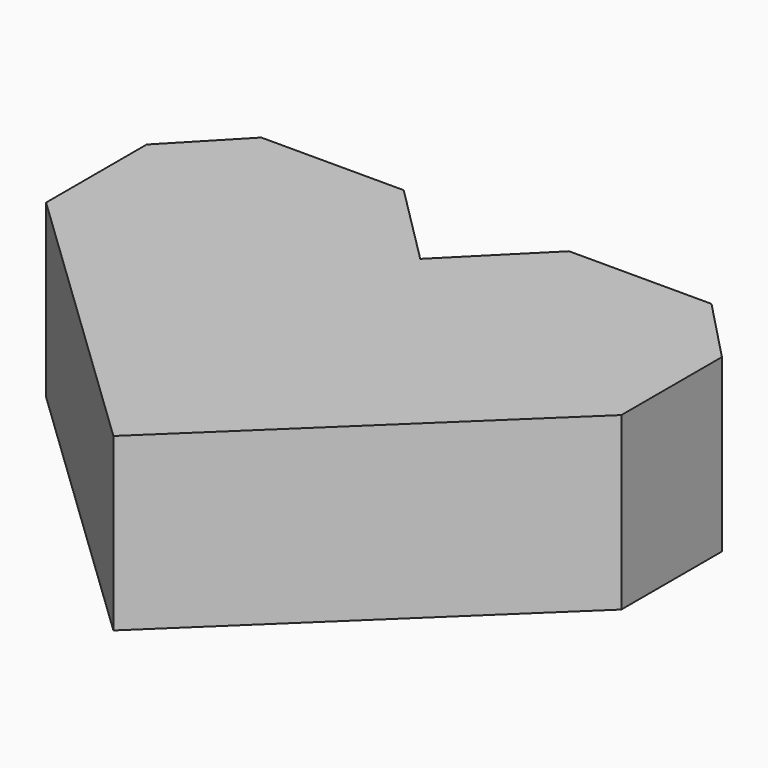
from build123d import *

# Parameters (mm, degrees)
F1_DEPTH = 25


# Not quite as in the source:
# - a feature names something its author has since deleted; it is built from what else it names


with BuildPart() as f1:
    # F0 (on Top) → F1 (new body)
    with BuildSketch(Plane.XY):
        Polygon((-41.9999984371, 3.9884479332), (-41.9999984371, -14.3649787007), (0, -54.5777431617), (41.9999984371, -14.3649787007), (41.9999984371, 3.9884479332), (32.8689099534, 13.4999984371), (12.0710684592, 13.4999984371), (0, 1.4289299778), (-12.0710684592, 13.4999984371), (-32.8689099534, 13.4999984371), align=None)
    extrude(amount=F1_DEPTH)


solid = f1.part
